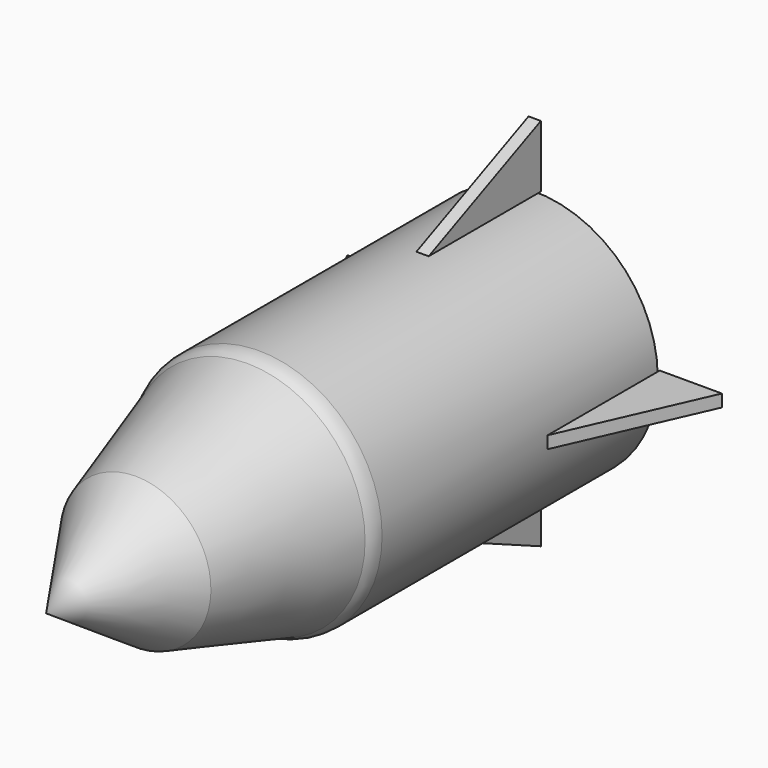
from build123d import *

# Parameters (mm, degrees)
F0_R            = 25.4
F1_DEPTH        = 76.2
F2_R            = 22.545291361
F3_DEPTH        = 69.342
F4_R            = 5.08
F8_DEPTH        = 1.27
F8_COPIES_COUNT = 4


# Not quite as in the source:
# - a pattern or mirror of a feature is missing from the dataset's text; its kind, count and spacing are read off the source's solid


with BuildPart() as f1:
    # F0 (on Front) → F1 (new body)
    with BuildSketch(Plane.XZ):
        Circle(F0_R)
    extrude(amount=F1_DEPTH)

    # F2 (on Front) → F3 (cut)
    with BuildSketch(Plane.XZ):
        Circle(F2_R)
    extrude(amount=F3_DEPTH, mode=Mode.SUBTRACT)

    # F4
    f4_edges = [f1.edges().sort_by_distance(p)[0] for p in [
        (-25.4, -76.2, 0),
    ]]
    fillet(f4_edges, radius=F4_R)

    # F5 (on Right) → F6 (revolve)
    with BuildSketch(Plane.YZ):
        Polygon((-126.0763704777, 0), (-71.3101625443, 0), (-71.3101625443, 25.2437964082), (-102.9718741775, 15.5456149951), align=None)
    revolve(axis=Axis((0, -98.693266511, 0), (0, -1, 0)))


with BuildPart() as f8:
    # F7 (on Right) → F8 (new body, symmetric)
    with BuildSketch(Plane.YZ):
        Polygon((0, 25.8142799139), (0, 38.6501066387), (-28.9315544069, 25.8142799139), align=None)
    extrude(amount=F8_DEPTH, both=True)


with BuildPart() as f8_copies_1:
    # F8_copies: instance of F8
    add(f8.part.rotate(Axis((0, 0, 0), (0, 1, 0)), 1 * 360 / F8_COPIES_COUNT))


with BuildPart() as f8_copies_2:
    # F8_copies: instance of F8
    add(f8.part.rotate(Axis((0, 0, 0), (0, 1, 0)), 2 * 360 / F8_COPIES_COUNT))


with BuildPart() as f8_copies_3:
    # F8_copies: instance of F8
    add(f8.part.rotate(Axis((0, 0, 0), (0, 1, 0)), 3 * 360 / F8_COPIES_COUNT))


solid = Compound([f1.part, f8.part, f8_copies_1.part, f8_copies_2.part, f8_copies_3.part])
